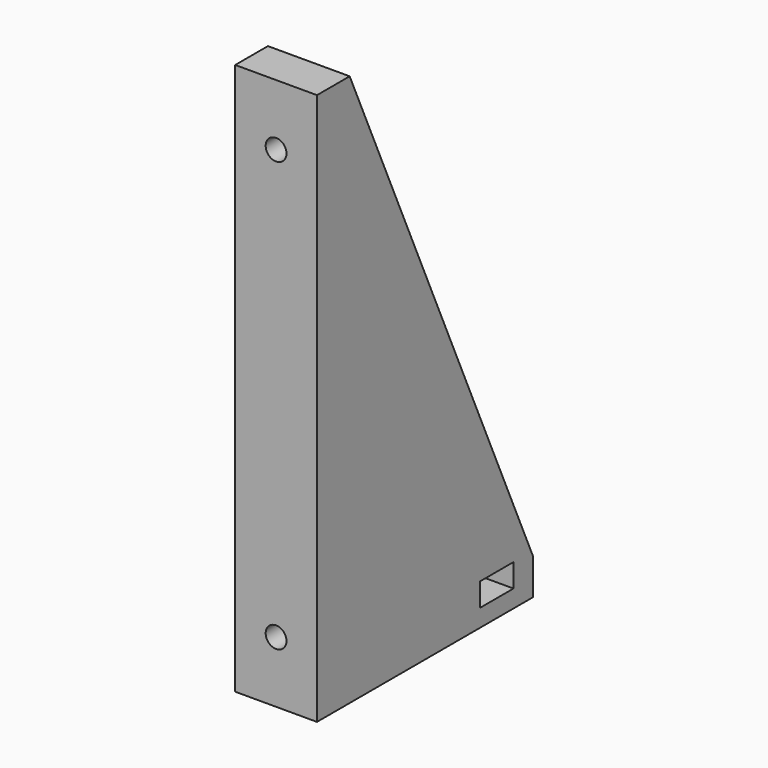
from build123d import *

# Parameters (mm, degrees)
F1_DEPTH  = 20
F3_D      = 5.1
F5_DEPTH  = 12
F6_DEPTH  = 25
F7_DEPTH  = 15
F8_D      = 5.1
F9_W      = 5.1
F9_H      = 5.7
F10_DEPTH = 25
F4_W      = 10
F4_H      = 4
F11_DEPTH = 25


# Not quite as in the source:
# - a feature names something its author has since deleted; it is built from what else it names


with BuildPart() as f1:
    # F0 (on Right) → F1 (new body)
    with BuildSketch(Plane.YZ):
        Polygon((-70, 0), (0, 0), (-60, 135), (-70, 135), align=None)
    extrude(amount=F1_DEPTH)

    # F3 (through all)
    with Locations(Plane.XZ.offset(70)):
        with Locations((10, 15), (10, 120)):
            Hole(F3_D / 2)

    # F4 (on face) → F5 (cut)
    with BuildSketch(Plane(origin=(0, 0, 0), x_dir=(1, 0, 0), z_dir=(0, 0, -1))):
        with BuildLine():
            ThreePointArc((12.55, 55), (11.803122292, 56.803122292), (10, 57.55))
            Line((10, 57.55), (10, 55))
            Line((10, 55), (10, 52.45))
            ThreePointArc((10, 52.45), (11.803122292, 53.196877708), (12.55, 55))
        make_face()
        with BuildLine():
            ThreePointArc((12.55, 15), (11.803122292, 16.803122292), (10, 17.55))
            ThreePointArc((10, 17.55), (8.196877708, 13.196877708), (12.55, 15))
        make_face()
        with BuildLine():
            Line((10, 55), (10, 57.55))
            ThreePointArc((10, 57.55), (7.45, 55), (10, 52.45))
            Line((10, 52.45), (10, 55))
        make_face()
    extrude(amount=-F5_DEPTH, mode=Mode.SUBTRACT)

    # F2 (on face) → F6 (join)
    with BuildSketch(Plane.XZ.offset(70)):
        Polygon((15.1, 122.9444863729), (10, 125.8889727457), (4.9, 122.9444863729), (4.9, 117.0555136271), (10, 114.1110272543), (15.1, 117.0555136271), align=None)
    extrude(amount=-F6_DEPTH)

    # F7 (cut): a face of the model
    f7_faces = [f1.faces().sort_by_distance(p)[0] for p in [
        (10, -45, 120),
    ]]
    extrude(f7_faces, amount=-F7_DEPTH, mode=Mode.SUBTRACT)

    # F8 (through all)
    with Locations(Plane.XZ.offset(70)):
        with Locations((10, 120)):
            Hole(F8_D / 2)

    # F9 (on face) → F10 (cut)
    with BuildSketch(Plane(origin=(0, 0, 0), x_dir=(0, -1, 0), z_dir=(-1, 0, 0))):
        with Locations((12.45, 7.15)):
            Rectangle(F9_W, F9_H)
        with Locations((17.55, 7.15)):
            Rectangle(F9_W, F9_H)
    extrude(amount=-F10_DEPTH, mode=Mode.SUBTRACT)

    # F4 (on face) → F11 (cut)
    with BuildSketch(Plane(origin=(0, 0, 0), x_dir=(1, 0, 0), z_dir=(0, 0, -1))):
        with Locations((15, 2)):
            Rectangle(F4_W, F4_H)
        with Locations((5, 2)):
            Rectangle(F4_W, F4_H)
    extrude(amount=-F11_DEPTH, mode=Mode.SUBTRACT)


solid = f1.part
